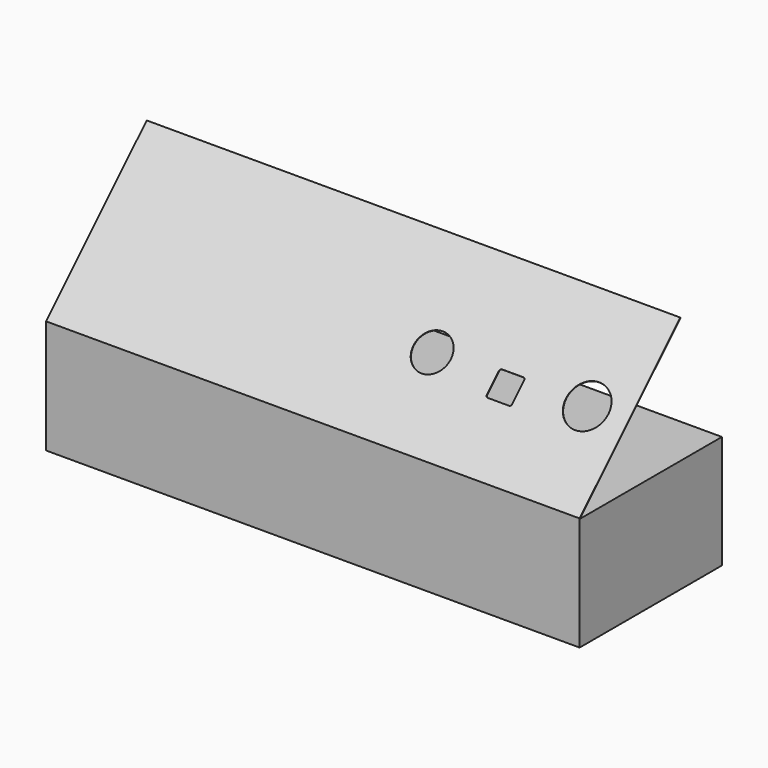
from build123d import *

# Parameters (mm, degrees)
F1_DEPTH = 209.55
F3_DEPTH = 0.4064


# Not quite as in the source:
# - the dataset's text gives a spline's control points without its knots; the knots are read off the source's solid


with BuildPart() as f1:
    # F0 (on Right) → F1 (new body, symmetric)
    with BuildSketch(Plane.YZ):
        Polygon((-139.7, 0), (0, 0), (0, 88.9), (-139.2936, 88.9), (-139.2936, 89.154), (-40.6298144724, 187.8177855276), (-40.9171826682, 188.1051537235), (-139.7, 89.3223363917), align=None)
    extrude(amount=F1_DEPTH, both=True)

    # F2 (on face) → F3 (cut, through all)
    with BuildSketch(Plane(origin=(0, -114.5111681959, 114.5111681959), x_dir=(1, 0, 0), z_dir=(0, -0.7071067812, 0.7071067812))):
        with BuildLine():
            add(Edge.make_bspline(
                [(107.5209936486, 34.5596805655), (107.2271156486, 34.2660057655), (107.0557164486, 33.8529255655), (107.0557164486, 33.4373053655)],
                knots=[1, 1, 1, 1, 2, 2, 2, 2], degree=3))
            Line((107.0557164486, 33.4373053655), (107.0557164486, 16.7685553655))
            add(Edge.make_bspline(
                [(107.0557164486, 16.7685553655), (107.0557164486, 16.3530875655), (107.2271156486, 15.9400073655), (107.5209936486, 15.6461547655)],
                knots=[0, 0, 0, 0, 1, 1, 1, 1], degree=3))
            add(Edge.make_bspline(
                [(107.5209936486, 15.6461547655), (107.8148462486, 15.3522767655), (108.2279264486, 15.1810553655), (108.6432164486, 15.1810553655)],
                knots=[1, 1, 1, 1, 2, 2, 2, 2], degree=3))
            Line((108.6432164486, 15.1810553655), (125.3119664486, 15.1810553655))
            add(Edge.make_bspline(
                [(125.3119664486, 15.1810553655), (125.7282978486, 15.1810553655), (126.1410224486, 15.3522767655), (126.4352306486, 15.6461547655)],
                knots=[0, 0, 0, 0, 1, 1, 1, 1], degree=3))
            add(Edge.make_bspline(
                [(126.4352306486, 15.6461547655), (126.7287784486, 15.9400073655), (126.8994664486, 16.3530875655), (126.8994664486, 16.7685553655)],
                knots=[1, 1, 1, 1, 2, 2, 2, 2], degree=3))
            Line((126.8994664486, 16.7685553655), (126.8994664486, 33.4373053655))
            add(Edge.make_bspline(
                [(126.8994664486, 33.4373053655), (126.8994664486, 33.8529255655), (126.7287784486, 34.2660057655), (126.4352306486, 34.5596805655)],
                knots=[0, 0, 0, 0, 1, 1, 1, 1], degree=3))
            add(Edge.make_bspline(
                [(126.4352306486, 34.5596805655), (126.1410224486, 34.8537363655), (125.7282978486, 35.0248053655), (125.3119664486, 35.0248053655)],
                knots=[1, 1, 1, 1, 2, 2, 2, 2], degree=3))
            Line((125.3119664486, 35.0248053655), (108.6432164486, 35.0248053655))
            add(Edge.make_bspline(
                [(108.6432164486, 35.0248053655), (108.2279264486, 35.0248053655), (107.8148462486, 34.8537363655), (107.5209936486, 34.5596805655)],
                knots=[0, 0, 0, 0, 1, 1, 1, 1], degree=3))
        make_face()
        with BuildLine():
            add(Edge.make_bspline(
                [(67.0366194486, 40.2491027655), (64.3180828486, 42.9673091655), (60.4971608486, 44.5497799655), (56.6525914486, 44.5497799655)],
                knots=[7, 7, 7, 7, 8, 8, 8, 8], degree=3))
            add(Edge.make_bspline(
                [(56.6525914486, 44.5497799655), (52.8087078486, 44.5497799655), (48.9877858486, 42.9673091655), (46.2695794486, 40.2491027655)],
                knots=[0, 0, 0, 0, 1, 1, 1, 1], degree=3))
            add(Edge.make_bspline(
                [(46.2695794486, 40.2491027655), (43.5510936486, 37.5305661655), (41.9682164486, 33.7101267655), (41.9682164486, 29.8654303655), (41.9682164486, 26.0211911655), (43.5510936486, 22.2004469655), (46.2695794486, 19.4822405655)],
                knots=[1, 1, 1, 1, 2, 2, 2, 3, 3, 3, 3], degree=3))
            add(Edge.make_bspline(
                [(46.2695794486, 19.4822405655), (48.9877858486, 16.7637039655), (52.8087078486, 15.1810553655), (56.6525914486, 15.1810553655), (60.4971608486, 15.1810553655), (64.3180828486, 16.7637039655), (67.0366194486, 19.4822405655)],
                knots=[3, 3, 3, 3, 4, 4, 4, 5, 5, 5, 5], degree=3))
            add(Edge.make_bspline(
                [(67.0366194486, 19.4822405655), (69.7551814486, 22.2004469655), (71.3369664486, 26.0211911655), (71.3369664486, 29.8654303655), (71.3369664486, 33.7101267655), (69.7551814486, 37.5305661655), (67.0366194486, 40.2491027655)],
                knots=[5, 5, 5, 5, 6, 6, 6, 7, 7, 7, 7], degree=3))
        make_face()
        with BuildLine():
            add(Edge.make_bspline(
                [(189.0894868486, 43.6364975655), (186.0037170486, 46.7222673655), (181.6666416486, 48.5185299655), (177.3027692486, 48.5185299655)],
                knots=[7, 7, 7, 7, 8, 8, 8, 8], degree=3))
            add(Edge.make_bspline(
                [(177.3027692486, 48.5185299655), (172.9388714486, 48.5185299655), (168.6018468486, 46.7222673655), (165.5164072486, 43.6364975655)],
                knots=[0, 0, 0, 0, 1, 1, 1, 1], degree=3))
            add(Edge.make_bspline(
                [(165.5164072486, 43.6364975655), (162.4309930486, 40.5507277655), (160.6340192486, 36.2136777655), (160.6340192486, 31.8498053655), (160.6340192486, 27.4859075655), (162.4309930486, 23.1488575655), (165.5164072486, 20.0630877655)],
                knots=[1, 1, 1, 1, 2, 2, 2, 3, 3, 3, 3], degree=3))
            add(Edge.make_bspline(
                [(165.5164072486, 20.0630877655), (168.6018468486, 16.9776735655), (172.9388714486, 15.1810553655), (177.3027692486, 15.1810553655), (181.6666416486, 15.1810553655), (186.0037170486, 16.9776735655), (189.0894868486, 20.0630877655)],
                knots=[3, 3, 3, 3, 4, 4, 4, 5, 5, 5, 5], degree=3))
            add(Edge.make_bspline(
                [(189.0894868486, 20.0630877655), (192.1752312486, 23.1488575655), (193.9715192486, 27.4859075655), (193.9715192486, 31.8498053655), (193.9715192486, 36.2136777655), (192.1752312486, 40.5507277655), (189.0894868486, 43.6364975655)],
                knots=[5, 5, 5, 5, 6, 6, 6, 7, 7, 7, 7], degree=3))
        make_face()
    extrude(amount=-F3_DEPTH, mode=Mode.SUBTRACT)


solid = f1.part
